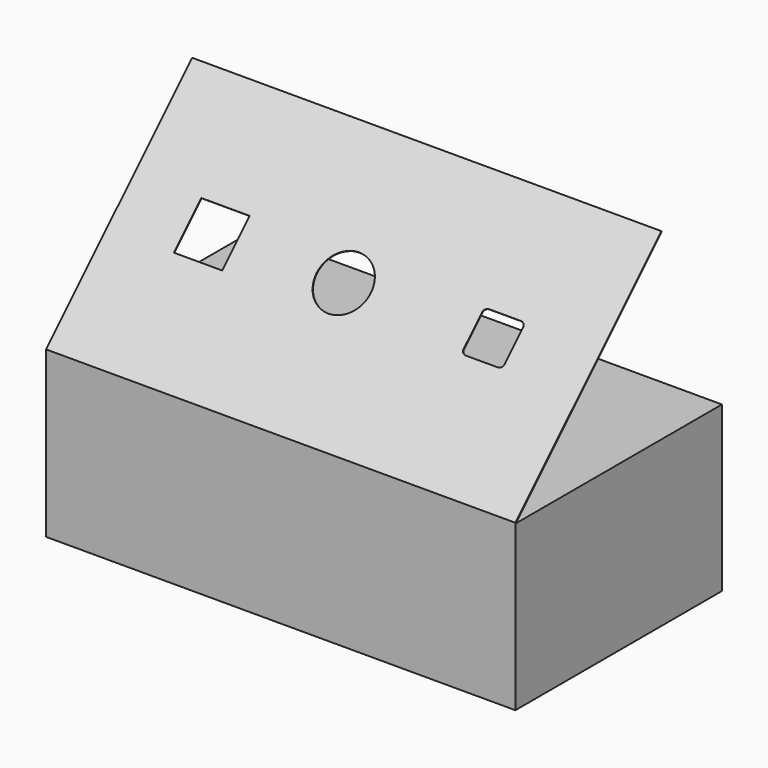
from build123d import *

# Parameters (mm, degrees)
F1_DEPTH = 127
F2_W     = 26.19375
F2_H     = 26.19375
F3_DEPTH = 0.4064


# Not quite as in the source:
# - the dataset's text gives a spline's control points without its knots; the knots are read off the source's solid


with BuildPart() as f1:
    # F0 (on Right) → F1 (new body, symmetric)
    with BuildSketch(Plane.YZ):
        Polygon((-139.7, 0), (0, 0), (0, 88.9), (-139.2936, 88.9), (-139.2936, 89.154), (-40.6298144724, 187.8177855276), (-40.9171826682, 188.1051537235), (-139.7, 89.3223363917), align=None)
    extrude(amount=F1_DEPTH, both=True)

    # F2 (on face) → F3 (cut, through all)
    with BuildSketch(Plane(origin=(0, -114.5111681959, 114.5111681959), x_dir=(1, 0, 0), z_dir=(0, -0.7071067812, 0.7071067812))):
        with Locations((-77.6792118578, 35.6651339804)):
            Rectangle(F2_W, F2_H)
        with BuildLine():
            add(Edge.make_bspline(
                [(64.3058991422, 46.0802007804), (63.8655901422, 45.6392313804), (63.6085929422, 45.0195983804), (63.6085929422, 44.3962315804)],
                knots=[1, 1, 1, 1, 2, 2, 2, 2], degree=3))
            Line((63.6085929422, 44.3962315804), (63.6085929422, 26.9337315804))
            add(Edge.make_bspline(
                [(63.6085929422, 26.9337315804), (63.6085929422, 26.3105171804), (63.8655901422, 25.6909095804), (64.3058991422, 25.2499401804)],
                knots=[0, 0, 0, 0, 1, 1, 1, 1], degree=3))
            add(Edge.make_bspline(
                [(64.3058991422, 25.2499401804), (64.7468685422, 24.8091485804), (65.3662983422, 24.5524815804), (65.9898429422, 24.5524815804)],
                knots=[1, 1, 1, 1, 2, 2, 2, 2], degree=3))
            Line((65.9898429422, 24.5524815804), (83.4523429422, 24.5524815804))
            add(Edge.make_bspline(
                [(83.4523429422, 24.5524815804), (84.0759129422, 24.5524815804), (84.6953681422, 24.8091485804), (85.1363375422, 25.2499401804)],
                knots=[0, 0, 0, 0, 1, 1, 1, 1], degree=3))
            add(Edge.make_bspline(
                [(85.1363375422, 25.2499401804), (85.5765957422, 25.6909095804), (85.8335929422, 26.3105171804), (85.8335929422, 26.9337315804)],
                knots=[1, 1, 1, 1, 2, 2, 2, 2], degree=3))
            Line((85.8335929422, 26.9337315804), (85.8335929422, 44.3962315804))
            add(Edge.make_bspline(
                [(85.8335929422, 44.3962315804), (85.8335929422, 45.0195983804), (85.5765957422, 45.6392313804), (85.1363375422, 46.0802007804)],
                knots=[0, 0, 0, 0, 1, 1, 1, 1], degree=3))
            add(Edge.make_bspline(
                [(85.1363375422, 46.0802007804), (84.6953681422, 46.5208145804), (84.0759129422, 46.7774815804), (83.4523429422, 46.7774815804)],
                knots=[1, 1, 1, 1, 2, 2, 2, 2], degree=3))
            Line((83.4523429422, 46.7774815804), (65.9898429422, 46.7774815804))
            add(Edge.make_bspline(
                [(65.9898429422, 46.7774815804), (65.3662983422, 46.7774815804), (64.7468685422, 46.5208145804), (64.3058991422, 46.0802007804)],
                knots=[0, 0, 0, 0, 1, 1, 1, 1], degree=3))
        make_face()
        with BuildLine():
            add(Edge.make_bspline(
                [(4.1421129422, 46.0483237804), (1.4239319422, 48.7668349804), (-2.3973710578, 50.3495089804), (-6.2414070578, 50.3495089804)],
                knots=[7, 7, 7, 7, 8, 8, 8, 8], degree=3))
            add(Edge.make_bspline(
                [(-6.2414070578, 50.3495089804), (-10.0854430578, 50.3495089804), (-13.9067460578, 48.7668349804), (-16.6249270578, 46.0483237804)],
                knots=[0, 0, 0, 0, 1, 1, 1, 1], degree=3))
            add(Edge.make_bspline(
                [(-16.6249270578, 46.0483237804), (-19.3434382578, 43.3299649804), (-20.9260868578, 39.5093477804), (-20.9260868578, 35.6649815804), (-20.9260868578, 31.8207677804), (-19.3434382578, 27.9999727804), (-16.6249270578, 25.2814615804)],
                knots=[1, 1, 1, 1, 2, 2, 2, 3, 3, 3, 3], degree=3))
            add(Edge.make_bspline(
                [(-16.6249270578, 25.2814615804), (-13.9067460578, 22.5629249804), (-10.0854430578, 20.9807589804), (-6.2414070578, 20.9807589804), (-2.3973710578, 20.9807589804), (1.4239319422, 22.5629249804), (4.1421129422, 25.2814615804)],
                knots=[3, 3, 3, 3, 4, 4, 4, 5, 5, 5, 5], degree=3))
            add(Edge.make_bspline(
                [(4.1421129422, 25.2814615804), (6.8610051422, 27.9999727804), (8.4429679422, 31.8207677804), (8.4429679422, 35.6649815804), (8.4429679422, 39.5093477804), (6.8610051422, 43.3299649804), (4.1421129422, 46.0483237804)],
                knots=[5, 5, 5, 5, 6, 6, 6, 7, 7, 7, 7], degree=3))
        make_face()
    extrude(amount=-F3_DEPTH, mode=Mode.SUBTRACT)


solid = f1.part
